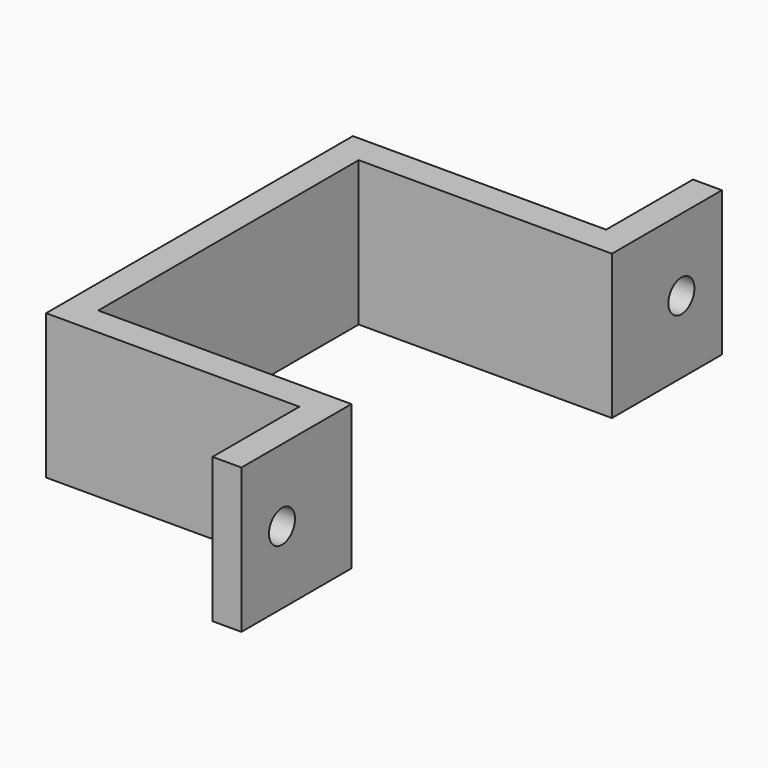
from build123d import *

# Parameters (mm, degrees)
F1_DEPTH = 20
F2_R     = 2.25
F3_DEPTH = 39.001


# Not quite as in the source:
# - a pattern or mirror of a feature is missing from the dataset's text; its kind, count and spacing are read off the source's solid


with BuildPart() as f1:
    # F0 (on Top) → F1 (new body)
    with BuildSketch(Plane.XY):
        Polygon((0, 26.5), (0, 0), (4, 0), (4, 22.5), (39, 22.5), (39, 41.5), (35, 41.5), (35, 26.5), align=None)
        Polygon((4, 0), (0, 0), (0, -26.5), (35, -26.5), (35, -41.5), (39, -41.5), (39, -22.5), (4, -22.5), align=None)
    extrude(amount=F1_DEPTH)

    # F2 (on Right) → F3 (cut, through all)
    with BuildSketch(Plane.YZ):
        with Locations((34.5, 10)):
            Circle(F2_R)
    f3 = extrude(amount=F3_DEPTH, mode=Mode.SUBTRACT)

    # F3_copies: F3 across plane
    add(f3.mirror(Plane(origin=(0, 0, 0), x_dir=(0, 0, -1), z_dir=(0, -1, 0))), mode=Mode.SUBTRACT)


solid = f1.part
